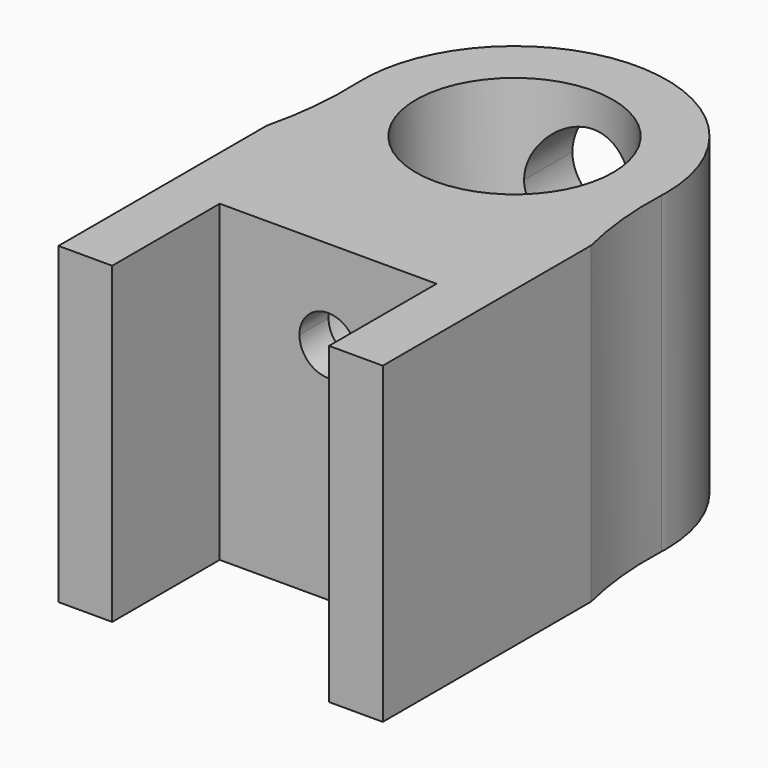
from build123d import *
from build123d import SkipClean  # not in build123d's __all__

# Parameters (mm, degrees)
F1_DEPTH    = 17.5
F2_DEPTH    = 9
F3_T4_DEPTH = 24.2978178738
F3_T9_DEPTH = 24.2978178738
F5_DEPTH    = 8.5
F6_DEPTH    = 25
F7_DEPTH    = 5
F8_DEPTH    = 25


# Not quite as in the source:
# - a fillet or chamfer that OpenCascade refuses, or shapes differently, is made with other operations: its cross-section is extruded or revolved along the edge and cut away or added
# - after a boolean that leaves OpenCascade's solid faulty, fix() repairs it
# - a feature names something its author has since deleted; it is built from what else it names


with BuildPart() as f1:
    # F0 (on Top) → F1 (new body)
    with BuildSketch(Plane.XY):
        Polygon((-6.05, -13), (-6.05, -5.9705527382), (-9.05, -5.9705527382), (-9.05, -20.5), (-6.05, -20.5), align=None)
        with BuildLine():
            Line((0, -13), (0, -8.5))
            ThreePointArc((0, -8.5), (-3.2787422684, -7.842183952), (-6.05, -5.9705527382))
            Line((-6.05, -5.9705527382), (-6.05, -13))
            Line((-6.05, -13), (0, -13))
        make_face()
        with BuildLine():
            ThreePointArc((6.05, -5.9705527382), (3.2787422684, -7.842183952), (0, -8.5))
            Line((0, -8.5), (0, -13))
            Line((0, -13), (6.05, -13))
            Line((6.05, -13), (6.05, -5.9705527382))
        make_face()
        Polygon((9.05, -5.9705527382), (6.05, -5.9705527382), (6.05, -13), (6.05, -20.5), (9.05, -20.5), align=None)
    extrude(amount=F1_DEPTH)

    # F0 (on Top) → F2 (join)
    with BuildSketch(Plane.XY):
        with BuildLine():
            Line((-6.05, -5.9705527382), (0, -5.9705527382))
            Line((0, -5.9705527382), (6.05, -5.9705527382))
            Line((6.05, -5.9705527382), (6.05, 5.9705527382))
            ThreePointArc((6.05, 5.9705527382), (0, 8.5), (-6.05, 5.9705527382))
            Line((-6.05, 5.9705527382), (-6.05, -5.9705527382))
        make_face()
        with BuildLine():
            ThreePointArc((0, -5.5), (-3.8890872965, 3.8890872965), (5.5, 0))
            ThreePointArc((5.5, 0), (3.8890872965, -3.8890872965), (0, -5.5))
        make_face(mode=Mode.SUBTRACT)
        with BuildLine():
            Line((6.05, 5.9705527382), (6.05, -5.9705527382))
            ThreePointArc((6.05, -5.9705527382), (7.8636823435, -3.2268405601), (8.5, 0))
            ThreePointArc((8.5, 0), (7.8636823435, 3.2268405601), (6.05, 5.9705527382))
        make_face()
        with BuildLine():
            ThreePointArc((-6.05, 5.9705527382), (-8.5, 0), (-6.05, -5.9705527382))
            Line((-6.05, -5.9705527382), (-6.05, 5.9705527382))
        make_face()
        with BuildLine():
            Line((0, -8.5), (0, -5.9705527382))
            Line((0, -5.9705527382), (-6.05, -5.9705527382))
            ThreePointArc((-6.05, -5.9705527382), (-3.2787422684, -7.842183952), (0, -8.5))
        make_face()
        with BuildLine():
            Line((6.05, -5.9705527382), (0, -5.9705527382))
            Line((0, -5.9705527382), (0, -8.5))
            ThreePointArc((0, -8.5), (3.2787422684, -7.842183952), (6.05, -5.9705527382))
        make_face()
    extrude(amount=F2_DEPTH)

    # F3: fillet of radius 20 on 4 edges, made by hand


with BuildPart() as f3_tool2:
    # F3_s3 → F3_t4 (new body)
    with BuildSketch(Plane.XY):
        with BuildLine():
            ThreePointArc((-9.05, -5.9705527382), (-8.5724849096, -3.1850150396), (-8.492373898, -0.3599799676))
            ThreePointArc((-8.492373898, -0.3599799676), (-7.7935737214, -3.3926698409), (-6.05, -5.9705527382))
            Line((-6.05, -5.9705527382), (-9.05, -5.9705527382))
        make_face()
    extrude(amount=F3_T4_DEPTH)

    split(bisect_by=Plane.XY.offset(17.5), keep=Keep.BOTTOM)


with BuildPart() as f1_1:
    add(f1.part, clean=False)

    # F3_t1: union F3_tool2
    add(f3_tool2.part)


with BuildPart() as f3_tool7:
    # F3_s8 → F3_t9 (new body)
    with BuildSketch(Plane.XY):
        with BuildLine():
            ThreePointArc((9.05, -5.9705527382), (8.5724849096, -3.1850150396), (8.492373898, -0.3599799676))
            ThreePointArc((8.492373898, -0.3599799676), (7.7935737214, -3.3926698409), (6.05, -5.9705527382))
            Line((6.05, -5.9705527382), (9.05, -5.9705527382))
        make_face()
    extrude(amount=F3_T9_DEPTH)

    split(bisect_by=Plane.XY.offset(17.5), keep=Keep.BOTTOM)


with BuildPart() as f1_2:
    add(f1_1.part, clean=False)

    # F3_t6: union F3_tool7
    add(f3_tool7.part)

    # F5 (add, through all): a face of the model
    f5_faces = [f1_2.faces().sort_by_distance(p)[0] for p in [
        (0, -8.2595836944, 9),
    ]]
    extrude(f5_faces, amount=F5_DEPTH)

    # F4 (on face) → F6 (cut)
    with BuildSketch(Plane(origin=(0, -5.9705527382, 0), x_dir=(-1, 0, 0), z_dir=(0, 1, 0))):
        with BuildLine():
            ThreePointArc((3.1, 12.5), (2.1920310217, 14.6920310217), (0, 15.6))
            ThreePointArc((0, 15.6), (-2.1920310217, 10.3079689783), (3.1, 12.5))
        make_face()
        with BuildLine():
            ThreePointArc((1.6, 12.5), (-1.1313708499, 11.3686291501), (0, 14.1))
            ThreePointArc((0, 14.1), (1.1313708499, 13.6313708499), (1.6, 12.5))
        make_face(mode=Mode.SUBTRACT)
        with BuildLine():
            ThreePointArc((1.6, 12.5), (1.1313708499, 13.6313708499), (0, 14.1))
            ThreePointArc((0, 14.1), (-1.1313708499, 11.3686291501), (1.6, 12.5))
        make_face()
    extrude(amount=F6_DEPTH, mode=Mode.SUBTRACT)

    # F4 (on face) → F7 (cut)
    with BuildSketch(Plane(origin=(0, -5.9705527382, 0), x_dir=(-1, 0, 0), z_dir=(0, 1, 0))):
        with BuildLine():
            ThreePointArc((3.1, 12.5), (2.1920310217, 14.6920310217), (0, 15.6))
            ThreePointArc((0, 15.6), (-2.1920310217, 10.3079689783), (3.1, 12.5))
        make_face()
        with BuildLine():
            ThreePointArc((1.6, 12.5), (-1.1313708499, 11.3686291501), (0, 14.1))
            ThreePointArc((0, 14.1), (1.1313708499, 13.6313708499), (1.6, 12.5))
        make_face(mode=Mode.SUBTRACT)
    with SkipClean():  # cleaning this boolean's faces spoils the solid; the shape is the same uncleaned
        extrude(amount=-F7_DEPTH, mode=Mode.SUBTRACT)

    # F4 (on face) → F8 (cut)
    with BuildSketch(Plane(origin=(0, -5.9705527382, 0), x_dir=(-1, 0, 0), z_dir=(0, 1, 0))):
        with BuildLine():
            ThreePointArc((1.6, 12.5), (1.1313708499, 13.6313708499), (0, 14.1))
            ThreePointArc((0, 14.1), (-1.1313708499, 11.3686291501), (1.6, 12.5))
        make_face()
    extrude(amount=-F8_DEPTH, mode=Mode.SUBTRACT)

    add(f1_2.part.fix(), mode=Mode.REPLACE)


solid = f1_2.part
